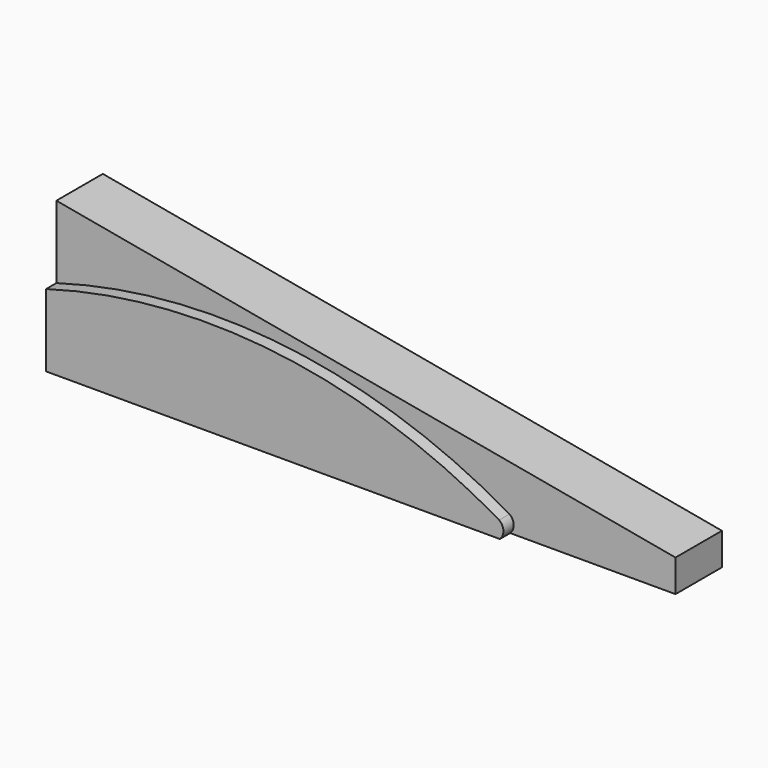
from build123d import *

# Parameters (mm, degrees)
F1_DEPTH = 41.275
F2_R     = 10.3124
F3_DEPTH = 50.8
F5_DEPTH = 6.35


# Not quite as in the source:
# - a pattern or mirror of a feature is missing from the dataset's text; its kind, count and spacing are read off the source's solid


with BuildPart() as f1:
    # F0 (on Front) → F1 (new body)
    with BuildSketch(Plane.XZ):
        Polygon((0, 71.4375), (0, 0), (304.8, 0), (304.8, 15.875), align=None)
    extrude(amount=F1_DEPTH)

    # F2 (on face) → F3 (cut)
    with BuildSketch(Plane(origin=(0, 0, 0), x_dir=(0, -1, 0), z_dir=(-1, 0, 0))):
        with Locations((20.6375, 32.5501)):
            Circle(F2_R)
    extrude(amount=-F3_DEPTH, mode=Mode.SUBTRACT)

    # F4 (on face) → F5 (cut)
    with BuildSketch(Plane.XZ.offset(41.275)):
        with BuildLine():
            Line((0, 71.4375), (0, 35.71875))
            ThreePointArc((0, 35.71875), (114.380623494, 44.8132958518), (223.1006332012, 8.1309120088))
            ThreePointArc((223.1006332012, 8.1309120088), (225.1513542681, 4.1369059415), (223.4067767859, 0))
            Line((223.4067767859, 0), (304.8, 0))
            Line((304.8, 0), (304.8, 7.9375))
            Line((304.8, 7.9375), (304.8, 15.875))
            Line((304.8, 15.875), (0, 71.4375))
        make_face()
    f5 = extrude(amount=-F5_DEPTH, mode=Mode.SUBTRACT)

    # F5_copies: F5 across plane
    add(f5.mirror(Plane.ZX.offset(-20.6375)), mode=Mode.SUBTRACT)


solid = f1.part
